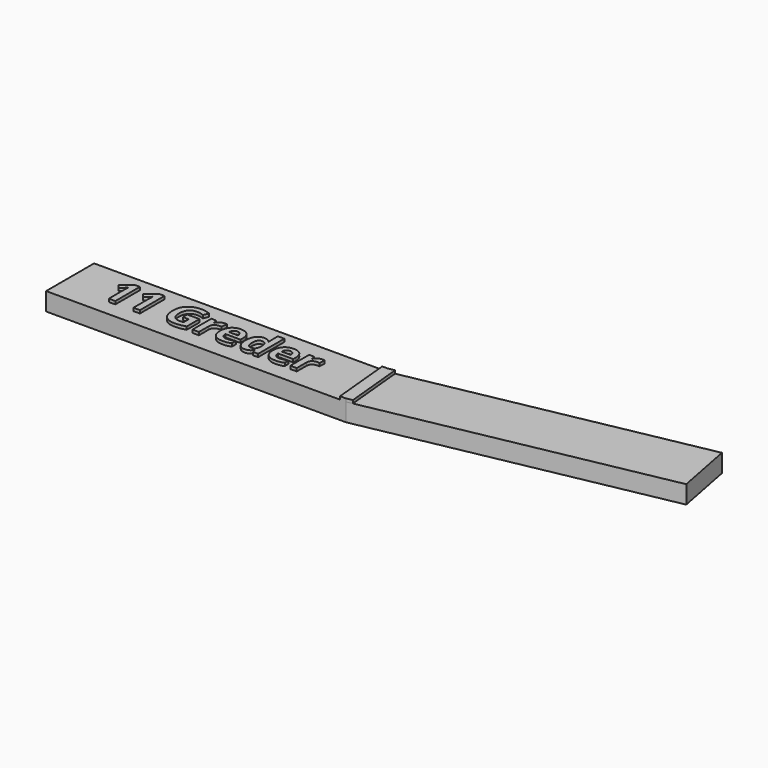
from build123d import *

# Parameters (mm, degrees)
F1_DEPTH     = 3
F2_TEXT_SIZE = 7.1878564389
F3_DEPTH     = 0.5


# Not quite as in the source:
# - Text() gives the source's letters only with a copy of the font that has no kerning and outlines rounded to 1/6400 em; it was checked with that copy


with BuildPart() as f1:
    # F0 (on Top) → F1 (new body)
    with BuildSketch(Plane.XY):
        Polygon((-50, 10), (-50, 0), (0, 0), (49.0813591724, 9.5404497688), (47.1732692186, 19.3567216033), (-0.962890482, 10), align=None)
    extrude(amount=F1_DEPTH)

    # F2 (on face) → F3 (join)
    with BuildSketch(Plane.XY.offset(3)):
        with Locations((-43.5774065554, 2.6826967951)):
            Text('11 Greder', F2_TEXT_SIZE, font='Open Sans', font_style=FontStyle.BOLD, text_align=(TextAlign.LEFT, TextAlign.BOTTOM))
        Polygon((0, 0), (-0.962890482, 10), (-1.9675155766, 10), (-1.9582866803, 9.9041542475), (-1.0046250947, 0), align=None)
        Polygon((0.0232768201, 10.191691505), (-0.962890482, 10), (0, 0), (0.9861673021, 0.191691505), (0.0325057164, 10.0958457525), align=None)
    extrude(amount=F3_DEPTH)


solid = f1.part
